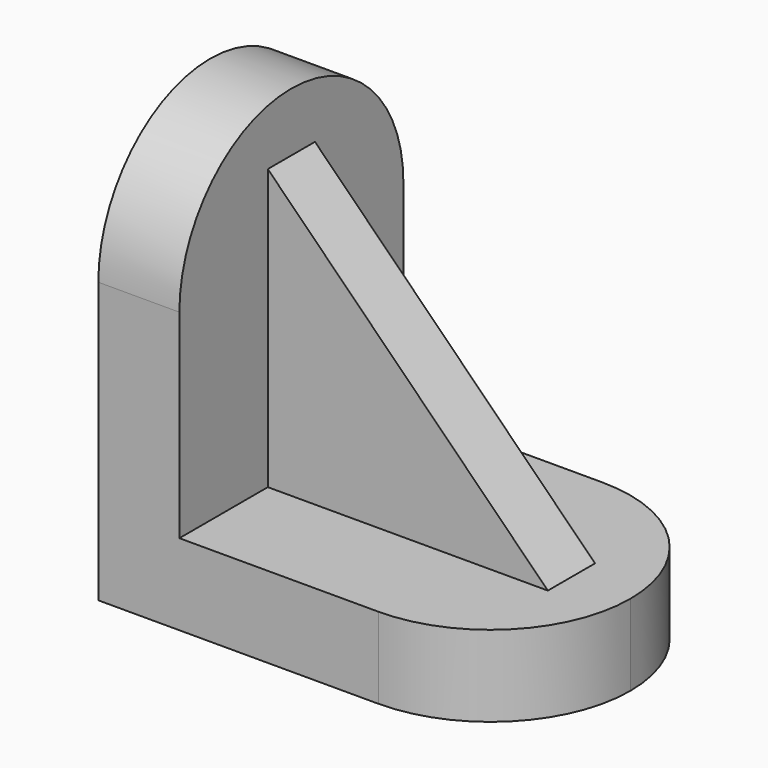
from build123d import *

# Parameters (mm, degrees)
F1_DEPTH  = 110
F2_W      = 110
F2_H      = 380
F3_DEPTH  = 270
F5_DEPTH  = 150
F7_DEPTH  = 150
F9_DEPTH  = 110
F10_W     = 80
F10_H     = 380
F11_DEPTH = 380
F13_DEPTH = 80


with BuildPart() as f1:
    # F0 (on Top) → F1 (new body)
    with BuildSketch(Plane.XY):
        with BuildLine():
            ThreePointArc((0, 380), (-190, 190), (0, 0))
            Line((0, 0), (0, 380))
        make_face()
        with BuildLine():
            Line((-380, 0), (0, 0))
            ThreePointArc((0, 0), (-190, 190), (0, 380))
            Line((0, 380), (-380, 380))
            Line((-380, 380), (-380, 0))
        make_face()
        with BuildLine():
            Line((0, 380), (0, 0))
            ThreePointArc((0, 0), (134.3502884254, 55.6497115746), (190, 190))
            ThreePointArc((190, 190), (134.3502884254, 324.3502884254), (0, 380))
        make_face()
    extrude(amount=F1_DEPTH)

    # F2 (on face) → F3 (join)
    with BuildSketch(Plane.XY.offset(110)):
        with Locations((-325, 190)):
            Rectangle(F2_W, F2_H)
    extrude(amount=F3_DEPTH)

    # F4 (on face) → F5 (cut)
    with BuildSketch(Plane.XZ):
        Polygon((0, 110), (-270, 380), (-270, 110), align=None)
    extrude(amount=-F5_DEPTH, mode=Mode.SUBTRACT)

    # F6 (on face) → F7 (cut)
    with BuildSketch(Plane(origin=(0, 380, 0), x_dir=(-1, 0, 0), z_dir=(0, 1, 0))):
        Polygon((270, 110), (270, 380), (0, 110), align=None)
    extrude(amount=-F7_DEPTH, mode=Mode.SUBTRACT)

    # F8 (on face) → F9 (join)
    with BuildSketch(Plane(origin=(-380, 0, 0), x_dir=(0, -1, 0), z_dir=(-1, 0, 0))):
        with BuildLine():
            Line((-380, 380), (0, 380))
            ThreePointArc((0, 380), (-190, 570), (-380, 380))
        make_face()
        with BuildLine():
            ThreePointArc((-380, 380), (-190, 190), (0, 380))
            Line((0, 380), (-380, 380))
        make_face()
    extrude(amount=-F9_DEPTH)

    # F10 (on face) → F11 (join)
    with BuildSketch(Plane.YZ.offset(-270)):
        with Locations((190, 300)):
            Rectangle(F10_W, F10_H)
    extrude(amount=F11_DEPTH)

    # F12 (on face) → F13 (cut)
    with BuildSketch(Plane.XZ.offset(-150)):
        Polygon((110, 490), (-270, 490), (110, 110), align=None)
    extrude(amount=-F13_DEPTH, mode=Mode.SUBTRACT)


solid = f1.part
